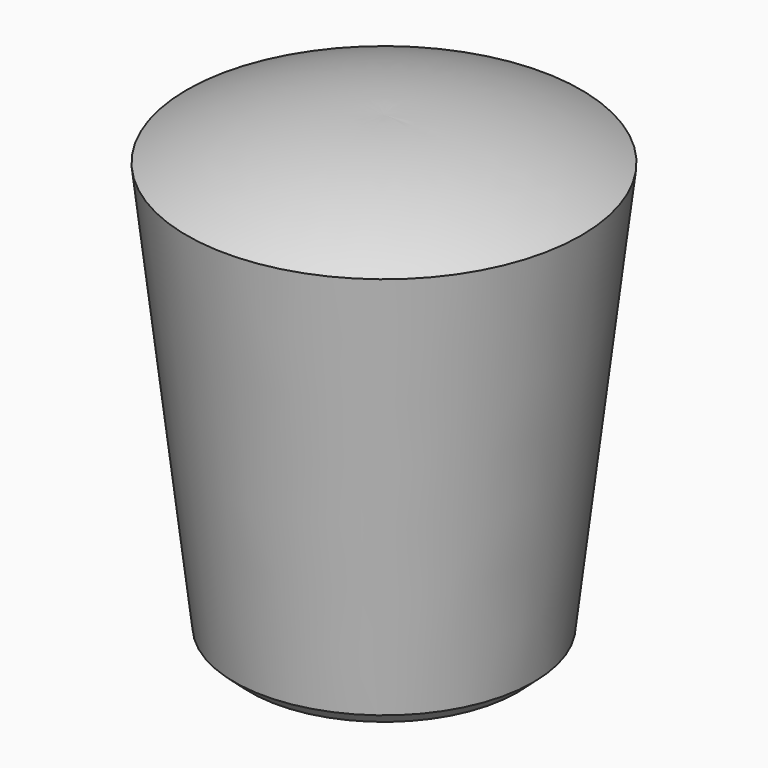
from build123d import *


# Not quite as in the source:
# - a fillet or chamfer that OpenCascade refuses, or shapes differently, is made with other operations: its cross-section is extruded or revolved along the edge and cut away or added


with BuildPart() as f1:
    # F0 (on Front) → F1 (revolve)
    with BuildSketch(Plane.XZ):
        with BuildLine():
            Line((0, 22), (0, 15))
            Line((0, 15), (1.5, 15))
            Line((1.5, 15), (1.5, 0))
            Line((1.5, 0), (7, 0))
            Line((7, 0), (9.3309248539, 20))
            ThreePointArc((9.3309248539, 20), (4.7864955847, 21.56467565), (0, 22))
        make_face()
    revolve(axis=Axis((0, 0, 17.1563792974), (0, 0, 1)))

    # F2: chamfer of 0.75 on 2 edges, made by hand

    # F2_s1 → F2_t2 (revolve, cut)
    with BuildSketch(Plane.XZ):
        Polygon((1.5, 0.75), (2.25, 0), (1.5, 0), align=None)
    revolve(axis=Axis((0, 0, 0), (0, 0, 1)), mode=Mode.SUBTRACT)

    # F2_s3 → F2_t4 (revolve, cut)
    with BuildSketch(Plane.XZ):
        Polygon((6.3323332273, 0), (7.077290902, 0.663177982), (7, 0), align=None)
    revolve(axis=Axis((0, 0, 0), (0, 0, 1)), mode=Mode.SUBTRACT)


solid = f1.part
